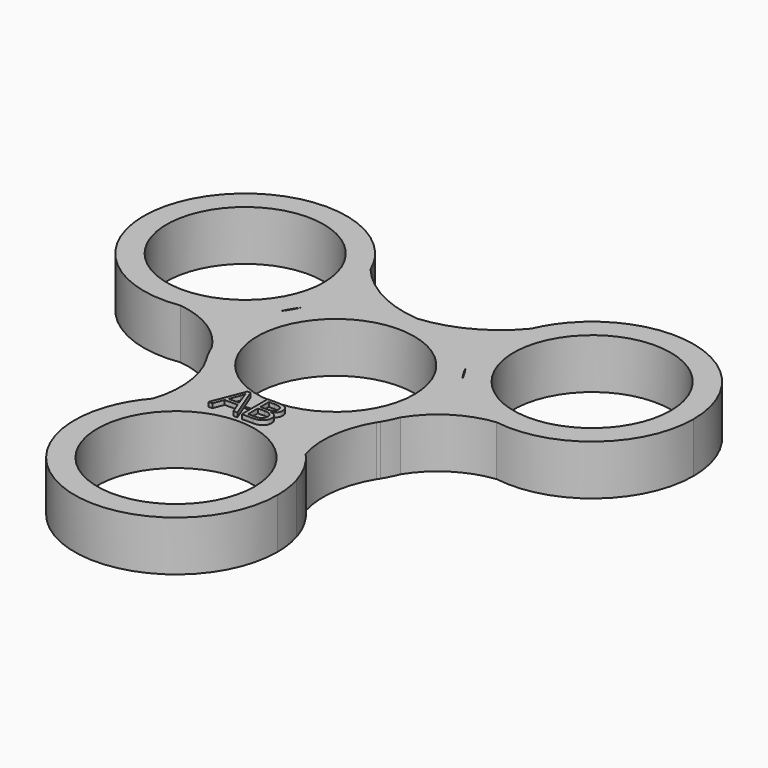
from build123d import *

# Parameters (mm, degrees)
F0_R         = 10.995861772
F1_DEPTH     = 7.0104
F2_TEXT_SIZE = 6.3621180339
F3_DEPTH     = 7.62


# Not quite as in the source:
# - Text() gives the source's letters only with a copy of the font that has no kerning and outlines rounded to 1/6400 em; it was checked with that copy


with BuildPart() as f1:
    # F0 (on Top) → F1 (new body)
    with BuildSketch(Plane.XY):
        with BuildLine():
            ThreePointArc((13.2269910459, -5.1688599841), (13.9554261685, -2.6299213143), (14.2010705816, 0))
            ThreePointArc((14.2010705816, 0), (13.8490275107, 3.1424262393), (12.8103525209, 6.1290516358))
            ThreePointArc((12.8103525209, 6.1290516358), (12.0870164452, 7.2218021007), (11.4674910141, 8.376577792))
            ThreePointArc((11.4674910141, 8.376577792), (6.4309421241, 12.6614923709), (0, 14.2010705816))
            ThreePointArc((0, 14.2010705816), (-6.4309421241, 12.6614923709), (-11.4674910141, 8.376577792))
            ThreePointArc((-11.4674910141, 8.376577792), (-12.0870164452, 7.2218021007), (-12.8103525209, 6.1290516358))
            ThreePointArc((-12.8103525209, 6.1290516358), (-14.1914240563, 0.5233439759), (-13.2269910459, -5.1688599841))
            ThreePointArc((-13.2269910459, -5.1688599841), (-12.6360938636, -6.230237361), (-12.1539315594, -7.3452265665))
            ThreePointArc((-12.1539315594, -7.3452265665), (-12.0634202818, -7.488971384), (-11.9747489071, -7.6338584133))
            ThreePointArc((-11.9747489071, -7.6338584133), (-7.9211323634, -11.7866902794), (-2.544731419, -13.9712113887))
            ThreePointArc((-2.544731419, -13.9712113887), (0, -13.7413521958), (2.544731419, -13.9712113887))
            ThreePointArc((2.544731419, -13.9712113887), (7.8637715318, -11.8250371229), (11.9000040144, -7.7498587162))
            ThreePointArc((11.9000040144, -7.7498587162), (12.0251628935, -7.5464099777), (12.1539315594, -7.3452265665))
            ThreePointArc((12.1539315594, -7.3452265665), (12.6360938636, -6.230237361), (13.2269910459, -5.1688599841))
        make_face()
        Circle(F0_R, mode=Mode.SUBTRACT)
        with BuildLine():
            ThreePointArc((12.8103525209, 6.1290516358), (13.8490275107, 3.1424262393), (14.2010705816, 0))
            ThreePointArc((14.2010705816, 0), (13.9554261685, -2.6299213143), (13.2269910459, -5.1688599841))
            ThreePointArc((13.2269910459, -5.1688599841), (17.0236902378, -1.3404833182), (22.1016048207, 0.4722980085))
            ThreePointArc((22.1016048207, 0.4722980085), (16.892888855, 2.3757963688), (12.8103525209, 6.1290516358))
        make_face()
        with BuildLine():
            ThreePointArc((11.4674910141, 8.376577792), (12.1908270898, 7.283827327), (12.8103525209, 6.1290516358))
            ThreePointArc((12.8103525209, 6.1290516358), (16.892888855, 2.3757963688), (22.1016048207, 0.4722980085))
            ThreePointArc((22.1016048207, 0.4722980085), (33.5181218338, 3.7219536804), (38.4789141165, 14.5056294277))
            ThreePointArc((38.4789141165, 14.5056294277), (29.2279063551, 27.8160495466), (13.5276567135, 23.7848475503))
            ThreePointArc((13.5276567135, 23.7848475503), (12.5018931215, 21.879366185), (11.2356417687, 20.1244708343))
            ThreePointArc((11.2356417687, 20.1244708343), (10.079537702, 14.2254203314), (11.4674910141, 8.376577792))
        make_face()
        with Locations((24.2778435349, 14.5056294277)):
            Circle(F0_R, mode=Mode.SUBTRACT)
        with BuildLine():
            ThreePointArc((12.1539315594, -7.3452265665), (12.7370306959, -6.2800043562), (13.2269910459, -5.1688599841))
            ThreePointArc((13.2269910459, -5.1688599841), (12.6360938636, -6.230237361), (12.1539315594, -7.3452265665))
        make_face()
        with BuildLine():
            ThreePointArc((0, 14.2010705816), (6.4309421241, 12.6614923709), (11.4674910141, 8.376577792))
            ThreePointArc((11.4674910141, 8.376577792), (10.079537702, 14.2254203314), (11.2356417687, 20.1244708343))
            ThreePointArc((11.2356417687, 20.1244708343), (6.2104468131, 16.0386642228), (0, 14.2010705816))
        make_face()
        with BuildLine():
            ThreePointArc((11.9000040144, -7.7498587162), (12.0286693337, -7.5486104498), (12.1539315594, -7.3452265665))
            ThreePointArc((12.1539315594, -7.3452265665), (12.0251628935, -7.5464099777), (11.9000040144, -7.7498587162))
        make_face()
        with BuildLine():
            ThreePointArc((-11.4674910141, 8.376577792), (-6.4309421241, 12.6614923709), (0, 14.2010705816))
            ThreePointArc((0, 14.2010705816), (-6.2104468131, 16.0386642228), (-11.2356417687, 20.1244708343))
            ThreePointArc((-11.2356417687, 20.1244708343), (-10.369507303, 17.3741811391), (-10.0767729534, 14.5056294277))
            ThreePointArc((-10.0767729534, 14.5056294277), (-10.4288160242, 11.3632031884), (-11.4674910141, 8.376577792))
        make_face()
        with BuildLine():
            ThreePointArc((13.5276567135, 23.7848475503), (12.2416884968, 22.0422982914), (11.2356417687, 20.1244708343))
            ThreePointArc((11.2356417687, 20.1244708343), (12.5018931215, 21.879366185), (13.5276567135, 23.7848475503))
        make_face()
        with BuildLine():
            ThreePointArc((10.5055733605, -18.3871449672), (10.090703686, -12.9227197899), (11.9000040144, -7.7498587162))
            ThreePointArc((11.9000040144, -7.7498587162), (7.8637715318, -11.8250371229), (2.544731419, -13.9712113887))
            ThreePointArc((2.544731419, -13.9712113887), (6.8885942725, -15.5239818684), (10.5055733605, -18.3871449672))
        make_face()
        with BuildLine():
            ThreePointArc((-12.8103525209, 6.1290516358), (-12.1908270898, 7.283827327), (-11.4674910141, 8.376577792))
            ThreePointArc((-11.4674910141, 8.376577792), (-10.4288160242, 11.3632031884), (-10.0767729534, 14.5056294277))
            ThreePointArc((-10.0767729534, 14.5056294277), (-10.369507303, 17.3741811391), (-11.2356417687, 20.1244708343))
            ThreePointArc((-11.2356417687, 20.1244708343), (-12.5018931215, 21.879366185), (-13.5276567135, 23.7848475503))
            ThreePointArc((-13.5276567135, 23.7848475503), (-37.6060790077, 19.4075213937), (-22.1016048207, 0.4722980085))
            ThreePointArc((-22.1016048207, 0.4722980085), (-16.892888855, 2.3757963688), (-12.8103525209, 6.1290516358))
        make_face()
        with Locations((-24.2778435349, 14.5056294277)):
            Circle(F0_R, mode=Mode.SUBTRACT)
        with BuildLine():
            ThreePointArc((-13.5276567135, 23.7848475503), (-12.5018931215, 21.879366185), (-11.2356417687, 20.1244708343))
            ThreePointArc((-11.2356417687, 20.1244708343), (-12.2416884968, 22.0422982914), (-13.5276567135, 23.7848475503))
        make_face()
        with BuildLine():
            ThreePointArc((10.5055733605, -18.3871449672), (6.8885942725, -15.5239818684), (2.544731419, -13.9712113887))
            ThreePointArc((2.544731419, -13.9712113887), (0, -14.2010705816), (-2.544731419, -13.9712113887))
            ThreePointArc((-2.544731419, -13.9712113887), (-7.0184962879, -15.5969330941), (-10.7037375155, -18.6096627965))
            ThreePointArc((-10.7037375155, -18.6096627965), (-11.8286173317, -21.15089336), (-13.4561748187, -23.4035060663))
            ThreePointArc((-13.4561748187, -23.4035060663), (-2.299817091, -41.9560321273), (14.2010705816, -27.9424227774))
            ThreePointArc((14.2010705816, -27.9424227774), (14.046264318, -25.8512832862), (13.585220622, -23.805734934))
            ThreePointArc((13.585220622, -23.805734934), (11.7256883863, -21.2781458438), (10.5055733605, -18.3871449672))
        make_face()
        with Locations((0, -27.9424227774)):
            Circle(F0_R, mode=Mode.SUBTRACT)
        with BuildLine():
            ThreePointArc((13.585220622, -23.805734934), (12.3463301424, -20.9254050577), (10.5055733605, -18.3871449672))
            ThreePointArc((10.5055733605, -18.3871449672), (11.7256883863, -21.2781458438), (13.585220622, -23.805734934))
        make_face()
        with BuildLine():
            ThreePointArc((-13.2269910459, -5.1688599841), (-14.1914240563, 0.5233439759), (-12.8103525209, 6.1290516358))
            ThreePointArc((-12.8103525209, 6.1290516358), (-16.892888855, 2.3757963688), (-22.1016048207, 0.4722980085))
            ThreePointArc((-22.1016048207, 0.4722980085), (-17.0236902378, -1.3404833182), (-13.2269910459, -5.1688599841))
        make_face()
        with BuildLine():
            ThreePointArc((-10.7037375155, -18.6096627965), (-7.0184962879, -15.5969330941), (-2.544731419, -13.9712113887))
            ThreePointArc((-2.544731419, -13.9712113887), (-7.9211323634, -11.7866902794), (-11.9747489071, -7.6338584133))
            ThreePointArc((-11.9747489071, -7.6338584133), (-10.1479009236, -12.9838017304), (-10.7037375155, -18.6096627965))
        make_face()
        with BuildLine():
            ThreePointArc((-12.1539315594, -7.3452265665), (-12.6360938636, -6.230237361), (-13.2269910459, -5.1688599841))
            ThreePointArc((-13.2269910459, -5.1688599841), (-12.7370306959, -6.2800043562), (-12.1539315594, -7.3452265665))
        make_face()
        with BuildLine():
            ThreePointArc((-12.1539315594, -7.3452265665), (-12.0652033696, -7.4900783249), (-11.9747489071, -7.6338584133))
            ThreePointArc((-11.9747489071, -7.6338584133), (-12.0634202818, -7.488971384), (-12.1539315594, -7.3452265665))
        make_face()
        with BuildLine():
            ThreePointArc((-13.4561748187, -23.4035060663), (-11.8286173317, -21.15089336), (-10.7037375155, -18.6096627965))
            ThreePointArc((-10.7037375155, -18.6096627965), (-12.315460784, -20.8713668917), (-13.4561748187, -23.4035060663))
        make_face()
    extrude(amount=F1_DEPTH)

    # F2 (on Top) → F3 (join)
    with BuildSketch(Plane.XY):
        with Locations((-4.7334162518, -16.3379199803)):
            Text('AB', F2_TEXT_SIZE, font='Open Sans', text_align=(TextAlign.LEFT, TextAlign.BOTTOM))
    extrude(amount=F3_DEPTH)


solid = f1.part
